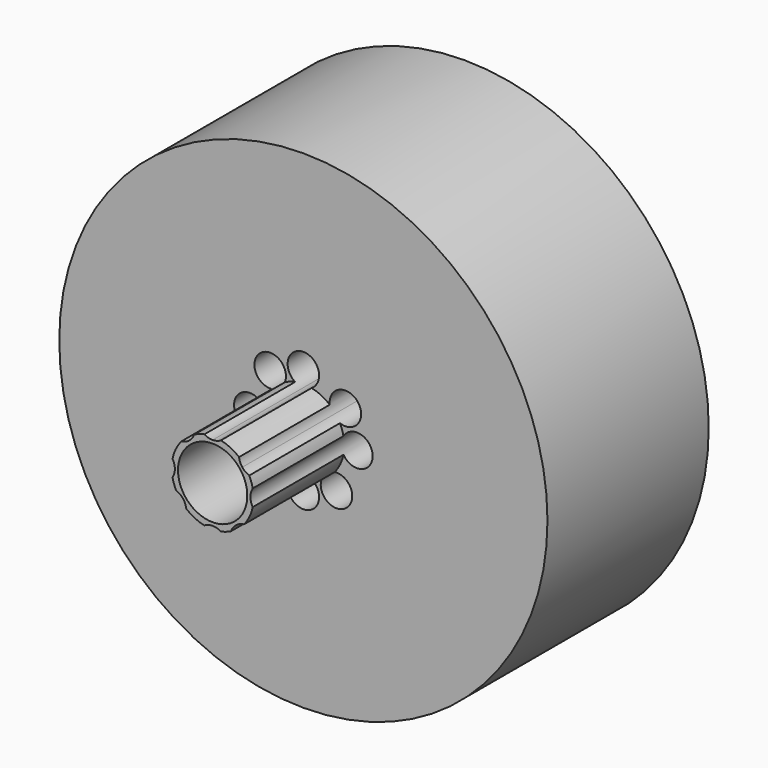
from build123d import *

# Parameters (mm, degrees)
F0_R     = 19.685
F1_DEPTH = 16.256
F2_R     = 8.382
F3_DEPTH = 12.7
F4_R     = 3.302
F5_DEPTH = 9.144
F6_R     = 1.27
F7_DEPTH = 25.4
F8_R     = 2.794
F9_DEPTH = 25.4


# Not quite as in the source:
# - a feature names something its author has since deleted; it is built from what else it names


with BuildPart() as f1:
    # F0 (on Front) → F1 (new body)
    with BuildSketch(Plane.XZ):
        Circle(F0_R)
    extrude(amount=F1_DEPTH)

    # F2 (on Front) → F3 (cut)
    with BuildSketch(Plane.XZ):
        Circle(F2_R)
    extrude(amount=F3_DEPTH, mode=Mode.SUBTRACT)

    # F4 (on face) → F5 (join)
    with BuildSketch(Plane.XZ.offset(16.256)):
        Circle(F4_R)
    extrude(amount=F5_DEPTH)

    # F6 (on Front) → F7 (cut)
    with BuildSketch(Plane.XZ):
        with BuildLine():
            ThreePointArc((1.27, 4.318), (-0.8980256121, 5.2160256121), (0, 3.048))
            ThreePointArc((0, 3.048), (0.8980256121, 3.4199743879), (1.27, 4.318))
        make_face()
        with BuildLine():
            ThreePointArc((-1.4060126705, 3.3888169304), (-3.8189189305, 3.9425906032), (-1.8889501203, 2.3921060685))
            ThreePointArc((-1.8889501203, 2.3921060685), (-1.5331064104, 2.8350432576), (-1.4060126705, 3.3888169304))
        make_face()
        with Locations((-4.318, 0)):
            Circle(F6_R)
        with BuildLine():
            ThreePointArc((-2.1188169304, -2.6760126705), (-2.1890830443, -2.259433023), (-2.3921060685, -1.8889501203))
            ThreePointArc((-2.3921060685, -1.8889501203), (-4.5885508164, -3.092592318), (-2.1188169304, -2.6760126705))
        make_face()
        with BuildLine():
            ThreePointArc((1.27, -4.318), (0.8980256121, -3.4199743879), (0, -3.048))
            ThreePointArc((0, -3.048), (-0.8980256121, -5.2160256121), (1.27, -4.318))
        make_face()
        with BuildLine():
            ThreePointArc((3.9398354632, -3.3809943125), (3.2236091359, -2.2380880524), (1.882772913, -2.3842834506))
            ThreePointArc((1.882772913, -2.3842834506), (2.1160617904, -4.5239005725), (3.9398354632, -3.3809943125))
        make_face()
        with BuildLine():
            ThreePointArc((5.588, 0), (4.318, 1.27), (3.048, 0))
            ThreePointArc((3.048, 0), (4.318, -1.27), (5.588, 0))
        make_face()
        with BuildLine():
            ThreePointArc((4.6588169304, 2.6760126705), (2.9722372829, 3.8757465565), (2.3921060685, 1.8889501203))
            ThreePointArc((2.3921060685, 1.8889501203), (3.8053965779, 1.4762787844), (4.6588169304, 2.6760126705))
        make_face()
    extrude(amount=F7_DEPTH, mode=Mode.SUBTRACT)

    # F8 (on face) → F9 (cut)
    with BuildSketch(Plane(origin=(0, -12.7, 0), x_dir=(-1, 0, 0), z_dir=(0, 1, 0))):
        Circle(F8_R)
    extrude(amount=-F9_DEPTH, mode=Mode.SUBTRACT)


solid = f1.part
